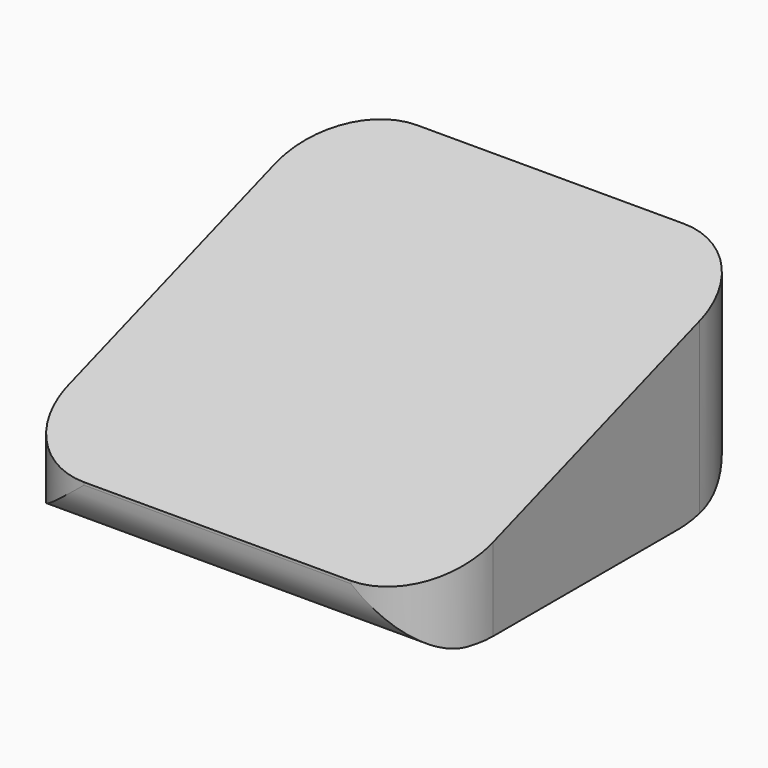
from build123d import *

# Parameters (mm, degrees)
F1_DEPTH    = 40.3
F2_R        = 15
F3_T1_DEPTH = 150.6
F4_T1_DEPTH = 100.6


# Not quite as in the source:
# - a fillet or chamfer that OpenCascade refuses, or shapes differently, is made with other operations: its cross-section is extruded or revolved along the edge and cut away or added


with BuildPart() as f1:
    # F0 (on Right) → F1 (new body, symmetric)
    with BuildSketch(Plane.YZ):
        Polygon((-39.5, 10.4954650627), (-39.5, 0), (39.5, 0), (39.5, 38), align=None)
    extrude(amount=F1_DEPTH, both=True)

    # F2
    f2_edges = [f1.edges().sort_by_distance(p)[0] for p in [
        (40.3, -39.5, 5.247733),
        (40.3, 39.5, 19),
        (-40.3, -39.5, 5.247733),
        (-40.3, 39.5, 19),
    ]]
    fillet(f2_edges, radius=F2_R)

    # F3: fillet of radius 20 on 1 edges, made by hand

    # F3_s2 → F3_t1 (cut)
    with BuildSketch(Plane.YZ.offset(-75.3)):
        with BuildLine():
            ThreePointArc((19.5, 0), (33.6421356237, 5.8578643763), (39.5, 20))
            Line((39.5, 20), (39.5, 0))
            Line((39.5, 0), (19.5, 0))
        make_face()
    extrude(amount=F3_T1_DEPTH, mode=Mode.SUBTRACT)

    # F4: fillet of radius 10 on 1 edges, made by hand

    # F4_s2 → F4_t1 (cut)
    with BuildSketch(Plane.YZ.offset(-50.3)):
        with BuildLine():
            ThreePointArc((-39.5, 10), (-36.5710678119, 2.9289321881), (-29.5, 0))
            Line((-29.5, 0), (-39.5, 0))
            Line((-39.5, 0), (-39.5, 10))
        make_face()
    extrude(amount=F4_T1_DEPTH, mode=Mode.SUBTRACT)


solid = f1.part
